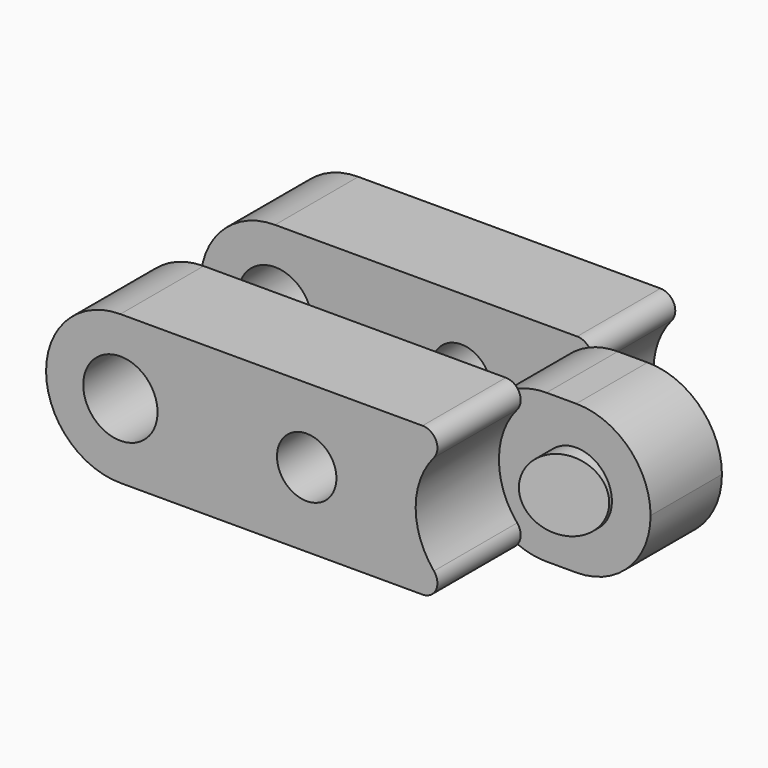
from build123d import *

# Parameters (mm, degrees)
F0_W         = 17.53
F0_H         = 10
F1_DEPTH     = 5
F3_DEPTH     = 10.001
F4_R         = 1.25
F5_DEPTH     = 10.001
F6_R         = 2.6
F7_DEPTH     = 3.5
F8_R         = 2.6
F9_DEPTH     = 3.5
F10_W        = 14.03
F10_H        = 3
F11_DEPTH    = 5.001
F12_R        = 1.2
F13_DEPTH    = 10
F14_R        = 0.5
F16_DEPTH    = 5.001
F17_T1_DEPTH = 3
F18_R        = 1
F19_DEPTH    = 10.001


# Not quite as in the source:
# - a fillet or chamfer that OpenCascade refuses, or shapes differently, is made with other operations: its cross-section is extruded or revolved along the edge and cut away or added


with BuildPart() as f1:
    # F0 (on Top) → F1 (new body)
    with BuildSketch(Plane.XY):
        Rectangle(F0_W, F0_H)
    extrude(amount=-F1_DEPTH)

    # F2 (on face) → F3 (cut, through all)
    with BuildSketch(Plane.XZ.offset(5)):
        with BuildLine():
            Line((8.765, 0), (6.265, 0))
            ThreePointArc((6.265, 0), (8.032766953, -0.732233047), (8.765, -2.5))
            Line((8.765, -2.5), (8.765, 0))
        make_face()
        with BuildLine():
            Line((8.765, -5), (8.765, -2.5))
            ThreePointArc((8.765, -2.5), (8.032766953, -4.267766953), (6.265, -5))
            Line((6.265, -5), (8.765, -5))
        make_face()
        with BuildLine():
            ThreePointArc((-6.265, -5), (-8.032766953, -4.267766953), (-8.765, -2.5))
            Line((-8.765, -2.5), (-8.765, -5))
            Line((-8.765, -5), (-6.265, -5))
        make_face()
        with BuildLine():
            ThreePointArc((-8.765, -2.5), (-8.032766953, -0.732233047), (-6.265, 0))
            Line((-6.265, 0), (-8.765, 0))
            Line((-8.765, 0), (-8.765, -2.5))
        make_face()
    extrude(amount=-F3_DEPTH, mode=Mode.SUBTRACT)

    # F4 (on face) → F5 (cut, through all)
    with BuildSketch(Plane(origin=(0, 5, 0), x_dir=(-1, 0, 0), z_dir=(0, 1, 0))):
        with Locations((6.265, -2.5)):
            Circle(F4_R)
    extrude(amount=-F5_DEPTH, mode=Mode.SUBTRACT)

    # F6 (on face) → F7 (cut)
    with BuildSketch(Plane(origin=(0, 5, 0), x_dir=(-1, 0, 0), z_dir=(0, 1, 0))):
        with Locations((-6.265, -2.5)):
            Circle(F6_R)
    extrude(amount=-F7_DEPTH, mode=Mode.SUBTRACT)

    # F8 (on face) → F9 (cut)
    with BuildSketch(Plane.XZ.offset(5)):
        with Locations((6.265, -2.5)):
            Circle(F8_R)
    extrude(amount=-F9_DEPTH, mode=Mode.SUBTRACT)

    # F10 (on face) → F11 (cut, through all)
    with BuildSketch(Plane.XY):
        with Locations((-4.25, 0)):
            Rectangle(F10_W, F10_H)
    extrude(amount=-F11_DEPTH, mode=Mode.SUBTRACT)

    # F12 (on face) → F13 (join)
    with BuildSketch(Plane(origin=(0, 5, 0), x_dir=(-1, 0, 0), z_dir=(0, 1, 0))):
        with Locations((-6.265, -2.5)):
            Circle(F12_R)
    extrude(amount=-F13_DEPTH)

    # F14
    f14_edges = [f1.edges().sort_by_distance(p)[0] for p in [
        (5.550857, 3.25, 0),
        (5.550857, -3.25, 0),
        (5.550857, -3.25, -5),
        (5.550857, 3.25, -5),
    ]]
    fillet(f14_edges, radius=F14_R)

    # F15 (on face) → F16 (cut, through all)
    with BuildSketch(Plane(origin=(0, 0, -5), x_dir=(1, 0, 0), z_dir=(0, 0, -1))):
        Polygon((8, 2.4762265265), (8, 5.5), (4.8, 5.5), (4.8, 2.5), (7.8, 1.5), align=None)
        Polygon((4.8, -5.5), (8, -5.5), (8, -2.4762265265), (7.8, -1.5), (4.8, -2.5), align=None)
    extrude(amount=-F16_DEPTH, mode=Mode.SUBTRACT)

    # F17: fillet of radius 2.5 on 2 edges, made by hand

    # F17_s2 → F17_t1 (cut)
    with BuildSketch(Plane.XZ.offset(-1.5)):
        with BuildLine():
            ThreePointArc((2.765, -2.5), (3.497233047, -0.732233047), (5.265, 0))
            Line((5.265, 0), (2.765, 0))
            Line((2.765, 0), (2.765, -2.5))
        make_face()
        with BuildLine():
            ThreePointArc((2.765, -2.5), (3.497233047, -4.267766953), (5.265, -5))
            Line((5.265, -5), (2.765, -5))
            Line((2.765, -5), (2.765, -2.5))
        make_face()
    extrude(amount=F17_T1_DEPTH, mode=Mode.SUBTRACT)

    # F18 (on face) → F19 (cut, through all)
    with BuildSketch(Plane.XZ.offset(5)):
        with Locations((0, -2.5)):
            Circle(F18_R)
    extrude(amount=-F19_DEPTH, mode=Mode.SUBTRACT)


solid = f1.part
